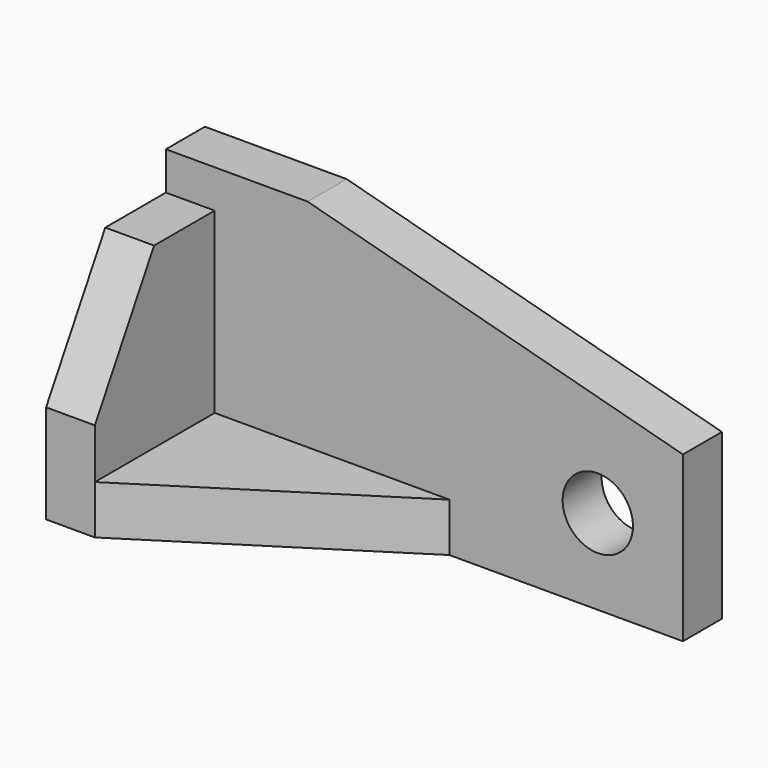
from build123d import *

# Parameters (mm, degrees)
F1_DEPTH = 10.922
F2_W     = 52.578
F2_H     = 10.922
F3_DEPTH = 33.528
F5_DEPTH = 10.923
F7_DEPTH = 115.7693519126
F8_R     = 7.874
F9_DEPTH = 10.923


# Not quite as in the source:
# - a feature names something its author has since deleted; it is built from what else it names


with BuildPart() as f1:
    # F0 (on Front) → F1 (new body)
    with BuildSketch(Plane.XZ):
        Polygon((-14.4320207924, 31.8836830556), (-46.1820207924, 31.8836830556), (-46.1820207924, -27.459501562), (-34.950372705, -27.459501562), (69.5863311203, -27.459501562), (69.5863311203, 9.3710335113), align=None)
    extrude(amount=-F1_DEPTH)

    # F2 (on face) → F3 (join)
    with BuildSketch(Plane.XZ):
        with Locations((-8.9710207924, -21.998501562)):
            Rectangle(F2_W, F2_H)
        Polygon((-35.2600207924, 23.340498438), (-46.1820207924, 23.340498438), (-46.1820207924, -27.459501562), (-35.2600207924, -27.459501562), (-35.2600207924, -16.537501562), align=None)
    extrude(amount=F3_DEPTH)

    # F4 (on face) → F5 (cut, through all)
    with BuildSketch(Plane.XY.offset(-16.537501562)):
        Polygon((17.3179792076, -33.528), (17.3179792076, 0), (-35.2600207924, -33.528), align=None)
    extrude(amount=-F5_DEPTH, mode=Mode.SUBTRACT)

    # F6 (on face) → F7 (cut, through all)
    with BuildSketch(Plane(origin=(-46.1820207924, 0, 0), x_dir=(0, -1, 0), z_dir=(-1, 0, 0))):
        Polygon((16.9568925737, 23.340498438), (33.528, -5.361501562), (33.528, 23.340498438), align=None)
    extrude(amount=-F7_DEPTH, mode=Mode.SUBTRACT)

    # F8 (on face) → F9 (cut, through all)
    with BuildSketch(Plane.XZ):
        with Locations((50.5363311203, -8.409501562)):
            Circle(F8_R)
    extrude(amount=-F9_DEPTH, mode=Mode.SUBTRACT)


solid = f1.part
